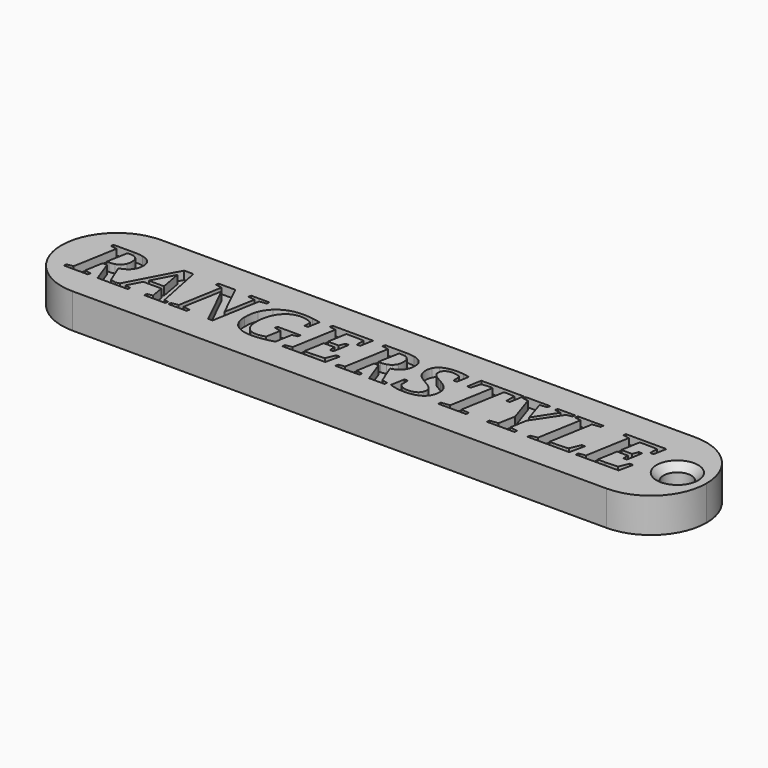
from build123d import *

# Parameters (mm, degrees)
F1_R     = 2
F2_DEPTH = 5
F3_START = 3.8
F3_DEPTH = 25
F4_SIZE  = 1


# Not quite as in the source:
# - ends of sketch curves that miss each other by under 0.0002 mm in the source are joined


with BuildPart() as f2:
    # F1 (on Top) → F2 (new body)
    with BuildSketch(Plane.XY):
        with BuildLine():
            Line((41.2404064533, 8), (-35.7595935467, 8))
            ThreePointArc((-35.7595935467, 8), (-41.4164477962, 5.6568542495), (-43.7595935467, 0))
            ThreePointArc((-43.7595935467, 0), (-41.4164477962, -5.6568542495), (-35.7595935467, -8))
            Line((-35.7595935467, -8), (41.2404064533, -8))
            ThreePointArc((41.2404064533, -8), (46.8972607028, -5.6568542495), (49.2404064533, 0))
            ThreePointArc((49.2404064533, 0), (46.8972607028, 5.6568542495), (41.2404064533, 8))
        make_face()
        with Locations((45.0494252145, 0)):
            Circle(F1_R, mode=Mode.SUBTRACT)
    extrude(amount=F2_DEPTH)

    # F0 (on Top) → F3 (cut)
    with BuildSketch(Plane.XY.offset(F3_START)):
        with BuildLine():
            add(Edge.make_bspline(
                [(-36.2724312993, 3.7303402653), (-35.7735742613, 3.7303402653), (-35.3449268567, 3.6896925164), (-34.9864890067, 3.6083970974)],
                knots=[0, 0, 0, 0, 1, 1, 1, 1], degree=3))
            Line((-36.2724312993, 3.7303402653), (-39.2378577235, 3.7303402653))
            Line((-39.2378577235, 3.7303402653), (-39.3099148564, 3.3257116948))
            Line((-39.3099148564, 3.3257116948), (-38.3842583864, 3.1815979019))
            Line((-38.3842583864, 3.1815979019), (-39.4983718703, -3.1483410183))
            Line((-39.4983718703, -3.1483410183), (-40.4073998198, -3.2979982558))
            Line((-40.4073998198, -3.2979982558), (-40.47391406, -3.7026261956))
            Line((-40.47391406, -3.7026261956), (-36.99854497, -3.7026261956))
            Line((-36.99854497, -3.7026261956), (-36.9320305721, -3.2979982558))
            Line((-36.9320305721, -3.2979982558), (-37.8576874363, -3.1483410183))
            Line((-37.8576874363, -3.1483410183), (-37.3976307265, -0.554285808))
            Line((-37.3976307265, -0.554285808), (-36.7546592649, -0.554285808))
            Line((-36.7546592649, -0.554285808), (-35.601745768, -3.7026261956))
            Line((-35.601745768, -3.7026261956), (-33.4622044537, -3.7026261956))
            Line((-33.4622044537, -3.7026261956), (-33.3846044279, -3.2979982558))
            Line((-33.3846044279, -3.2979982558), (-33.3572007613, -3.2908147575))
            Line((-33.3572007613, -3.2908147575), (-34.1328899849, -3.1483410183))
            Line((-34.1328899849, -3.1483410183), (-35.2470031536, -0.3990857565))
            add(Edge.make_bspline(
                [(-34.5264322969, -0.11085754), (-34.7481465097, -0.2328003137), (-34.9883368216, -0.3288763596), (-35.2470031536, -0.3990857565)],
                knots=[0, 0, 0, 0, 1, 1, 1, 1], degree=3))
            add(Edge.make_bspline(
                [(-33.9444330499, 0.3491998005), (-34.1070230995, 0.1681332577), (-34.3010228485, 0.0147808634), (-34.5264322969, -0.11085754)],
                knots=[0, 0, 0, 0, 1, 1, 1, 1], degree=3))
            add(Edge.make_bspline(
                [(-33.5619757351, 0.9977134454), (-33.654356782, 0.7501327412), (-33.7818426061, 0.5339615), (-33.9444330499, 0.3491998005)],
                knots=[0, 0, 0, 0, 1, 1, 1, 1], degree=3))
            add(Edge.make_bspline(
                [(-33.4234047561, 1.8568559118), (-33.4234047561, 1.5353701809), (-33.4695950825, 1.2489893851), (-33.5619757351, 0.9977134454)],
                knots=[0, 0, 0, 0, 1, 1, 1, 1], degree=3))
            add(Edge.make_bspline(
                [(-33.5896904355, 2.671655236), (-33.4788332896, 2.4388553953), (-33.4234047561, 2.1672556205), (-33.4234047561, 1.8568559118)],
                knots=[0, 0, 0, 0, 1, 1, 1, 1], degree=3))
            add(Edge.make_bspline(
                [(-34.1051752846, 3.253654483), (-33.8723754439, 3.0984548257), (-33.7005471083, 2.9044550767), (-33.5896904355, 2.671655236)],
                knots=[0, 0, 0, 0, 1, 1, 1, 1], degree=3))
            add(Edge.make_bspline(
                [(-34.9864890067, 3.6083970974), (-34.6280511567, 3.5307973082), (-34.3342799686, 3.4125497701), (-34.1051752846, 3.253654483)],
                knots=[0, 0, 0, 0, 1, 1, 1, 1], degree=3))
        make_face()
        with BuildLine():
            add(Edge.make_bspline(
                [(-36.9874593421, 0.0554281393), (-36.6844501044, 0.0554281393), (-36.4128503297, 0.094228231), (-36.1726600178, 0.1718284933)],
                knots=[0, 0, 0, 0, 1, 1, 1, 1], degree=3))
            Line((-36.9874593421, 0.0554281393), (-37.2923160004, 0.0554281393))
            Line((-37.2923160004, 0.0554281393), (-36.7491164509, 3.120626318))
            Line((-36.7491164509, 3.120626318), (-36.3666597669, 3.120626318))
            add(Edge.make_bspline(
                [(-35.3855747633, 2.8046834011), (-35.6072889761, 3.015311986), (-35.9343173632, 3.120626318), (-36.3666597669, 3.120626318)],
                knots=[0, 0, 0, 0, 1, 1, 1, 1], degree=3))
            add(Edge.make_bspline(
                [(-35.0474605907, 1.7681702582), (-35.0474605907, 2.248550803), (-35.1601653149, 2.5940552103), (-35.3855747633, 2.8046834011)],
                knots=[0, 0, 0, 0, 1, 1, 1, 1], degree=3))
            add(Edge.make_bspline(
                [(-35.1804893864, 1.0420559569), (-35.0918034963, 1.2563797774), (-35.0474605907, 1.4984179041), (-35.0474605907, 1.7681702582)],
                knots=[0, 0, 0, 0, 1, 1, 1, 1], degree=3))
            add(Edge.make_bspline(
                [(-35.5629460705, 0.5043992213), (-35.3966603911, 0.6522088805), (-35.2691748035, 0.831427766), (-35.1804893864, 1.0420559569)],
                knots=[0, 0, 0, 0, 1, 1, 1, 1], degree=3))
            add(Edge.make_bspline(
                [(-36.1726600178, 0.1718284933), (-35.932469706, 0.2494282825), (-35.7292317498, 0.3602851919), (-35.5629460705, 0.5043992213)],
                knots=[0, 0, 0, 0, 1, 1, 1, 1], degree=3))
        make_face(mode=Mode.SUBTRACT)
        Polygon((-32.8136908088, -3.1483410183), (-33.3572007613, -3.2908147575), (-33.3180906607, -3.2979982558), (-33.3846044279, -3.7026261956), (-31.2783206278, -3.7026261956), (-31.2007206021, -3.2979982558), (-32.0210627402, -3.1483410183), (-31.0011774085, -1.2249707087), (-28.3849509425, -1.2249707087), (-28.0468367699, -3.1483410183), (-28.8117507687, -3.2979982558), (-28.8893507944, -3.7026261956), (-25.8463238716, -3.7026261956), (-25.7687238458, -3.2979982558), (-26.3728949793, -3.1483410183), (-27.780779809, 3.7913112186), (-29.1110646131, 3.7913112186), align=None)
        Polygon((-30.6907779362, -0.6152567613), (-29.0556358431, 2.4942839288), (-28.4958078518, -0.6152567613), align=None, mode=Mode.SUBTRACT)
        Polygon((-33.3180906607, -3.2979982558), (-33.3572007613, -3.2908147575), (-33.3846044279, -3.2979982558), (-33.4622044537, -3.7026261956), (-33.3846044279, -3.7026261956), align=None)
        with BuildLine():
            add(Edge.make_bspline(
                [(-16.7006159225, -0.8037136964), (-16.7006159225, -0.0609715839), (-16.5805208059, 0.5967802681), (-16.3403304941, 1.1695419387)],
                knots=[0, 0, 0, 0, 1, 1, 1, 1], degree=3))
            add(Edge.make_bspline(
                [(-16.4844442871, -2.0619419193), (-16.6285583165, -1.6887228117), (-16.7006152918, -1.2693134566), (-16.7006159225, -0.8037136964)],
                knots=[0, 0, 0, 0, 1, 1, 1, 1], degree=3))
            add(Edge.make_bspline(
                [(-15.852559084, -3.0097694086), (-16.1297014361, -2.747407841), (-16.3403298635, -2.4314653971), (-16.4844442871, -2.0619419193)],
                knots=[0, 0, 0, 0, 1, 1, 1, 1], degree=3))
            add(Edge.make_bspline(
                [(-14.8215881243, -3.6083977281), (-15.2280641155, -3.4679789342), (-15.571721102, -3.2684361348), (-15.852559084, -3.0097694086)],
                knots=[0, 0, 0, 0, 1, 1, 1, 1], degree=3))
            add(Edge.make_bspline(
                [(-13.4192461084, -3.813483105), (-13.9439696378, -3.813483105), (-14.4114169764, -3.7451212864), (-14.8215881243, -3.6083977281)],
                knots=[0, 0, 0, 0, 1, 1, 1, 1], degree=3))
            add(Edge.make_bspline(
                [(-12.5545608281, -3.7802262214), (-12.8280084178, -3.8023974771), (-13.1162368708, -3.813483105), (-13.4192461084, -3.813483105)],
                knots=[0, 0, 0, 0, 1, 1, 1, 1], degree=3))
            add(Edge.make_bspline(
                [(-11.7563899457, -3.6804549399), (-12.0113615151, -3.7247978455), (-12.277418476, -3.7580549656), (-12.5545608281, -3.7802262214)],
                knots=[0, 0, 0, 0, 1, 1, 1, 1], degree=3))
            add(Edge.make_bspline(
                [(-11.0025622054, -3.5252548884), (-11.246447674, -3.5843786575), (-11.4977236137, -3.6361120343), (-11.7563899457, -3.6804549399)],
                knots=[0, 0, 0, 0, 1, 1, 1, 1], degree=3))
            add(Edge.make_bspline(
                [(-10.2653629069, -3.3146266976), (-10.512943611, -3.3922264869), (-10.7586767368, -3.4624358838), (-11.0025622054, -3.5252548884)],
                knots=[0, 0, 0, 0, 1, 1, 1, 1], degree=3))
            Line((-10.2653629069, -3.3146266976), (-9.8385630807, -0.8979421639))
            Line((-9.8385630807, -0.8979421639), (-9.0847347097, -0.7205708567))
            Line((-9.0847347097, -0.7205708567), (-9.0182209425, -0.3436569865))
            Line((-9.0182209425, -0.3436569865), (-12.3328470095, -0.3436569865))
            Line((-12.3328470095, -0.3436569865), (-12.3993614073, -0.7205708567))
            Line((-12.3993614073, -0.7205708567), (-11.4737045431, -0.8979421639))
            Line((-11.4737045431, -0.8979421639), (-11.8506184132, -3.0042265947))
            add(Edge.make_bspline(
                [(-12.3938185934, -3.1649694601), (-12.1610187527, -3.1095409266), (-11.9799519734, -3.0559599714), (-11.8506184132, -3.0042265947)],
                knots=[0, 0, 0, 0, 1, 1, 1, 1], degree=3))
            add(Edge.make_bspline(
                [(-13.1642747755, -3.2425694858), (-12.879741558, -3.2425694858), (-12.6229228044, -3.2167028368), (-12.3938185934, -3.1649694601)],
                knots=[0, 0, 0, 0, 1, 1, 1, 1], degree=3))
            add(Edge.make_bspline(
                [(-13.9014747047, -3.0984550622), (-13.6797604918, -3.1945313446), (-13.4340271295, -3.2425694858), (-13.1642747755, -3.2425694858)],
                knots=[0, 0, 0, 0, 1, 1, 1, 1], degree=3))
            add(Edge.make_bspline(
                [(-14.4723883238, -2.6661124221), (-14.3134930368, -2.8582649869), (-14.1231885233, -3.002379174), (-13.9014747047, -3.0984550622)],
                knots=[0, 0, 0, 0, 1, 1, 1, 1], degree=3))
            add(Edge.make_bspline(
                [(-14.84375938, -1.9344559375), (-14.7550739629, -2.2263795473), (-14.6312836109, -2.4702650947), (-14.4723883238, -2.6661124221)],
                knots=[0, 0, 0, 0, 1, 1, 1, 1], degree=3))
            add(Edge.make_bspline(
                [(-14.9767881758, -0.9145712364), (-14.9767881758, -1.3025707344), (-14.9324452701, -1.6425323277), (-14.84375938, -1.9344559375)],
                knots=[0, 0, 0, 0, 1, 1, 1, 1], degree=3))
            add(Edge.make_bspline(
                [(-14.7273596568, 0.8646846497), (-14.8936453361, 0.3473519856), (-14.9767881758, -0.2457332834), (-14.9767881758, -0.9145712364)],
                knots=[0, 0, 0, 0, 1, 1, 1, 1], degree=3))
            add(Edge.make_bspline(
                [(-14.0455884976, 2.1617125701), (-14.3301217151, 1.814360348), (-14.5573787419, 1.3820177078), (-14.7273596568, 0.8646846497)],
                knots=[0, 0, 0, 0, 1, 1, 1, 1], degree=3))
            add(Edge.make_bspline(
                [(-13.0589606801, 2.9598834525), (-13.4321793147, 2.7788169098), (-13.7610552801, 2.512759949), (-14.0455884976, 2.1617125701)],
                knots=[0, 0, 0, 0, 1, 1, 1, 1], degree=3))
            add(Edge.make_bspline(
                [(-11.8727902996, 3.2314832273), (-12.2866566831, 3.2314832273), (-12.6820468099, 3.1409499953), (-13.0589606801, 2.9598834525)],
                knots=[0, 0, 0, 0, 1, 1, 1, 1], degree=3))
            add(Edge.make_bspline(
                [(-10.8695334097, 3.0984550622), (-11.165152255, 3.1871404793), (-11.4995711921, 3.2314832273), (-11.8727902996, 3.2314832273)],
                knots=[0, 0, 0, 0, 1, 1, 1, 1], degree=3))
            add(Edge.make_bspline(
                [(-10.0990772275, 2.7270833753), (-10.3134006539, 2.8896738191), (-10.5702193287, 3.0134644077), (-10.8695334097, 3.0984550622)],
                knots=[0, 0, 0, 0, 1, 1, 1, 1], degree=3))
            Line((-10.0990772275, 2.7270833753), (-10.1046206721, 1.7626274442))
            Line((-10.1046206721, 1.7626274442), (-9.6390211484, 1.7626274442))
            Line((-9.6390211484, 1.7626274442), (-9.3341638594, 3.4698261184))
            add(Edge.make_bspline(
                [(-10.564677382, 3.7192546374), (-10.1397253706, 3.6601308684), (-9.7295542227, 3.5769880287), (-9.3341638594, 3.4698261184)],
                knots=[0, 0, 0, 0, 1, 1, 1, 1], degree=3))
            add(Edge.make_bspline(
                [(-11.9670193978, 3.813483105), (-11.4570767319, 3.813483105), (-10.9896293933, 3.7820736421), (-10.564677382, 3.7192546374)],
                knots=[0, 0, 0, 0, 1, 1, 1, 1], degree=3))
            add(Edge.make_bspline(
                [(-13.8349609374, 3.508625816), (-13.2585041102, 3.7118640086), (-12.6358568778, 3.813483105), (-11.9670193978, 3.813483105)],
                knots=[0, 0, 0, 0, 1, 1, 1, 1], degree=3))
            add(Edge.make_bspline(
                [(-15.3370742348, 2.616226466), (-14.9121222234, 3.0079215937), (-14.4114177647, 3.3053880175), (-13.8349609374, 3.508625816)],
                knots=[0, 0, 0, 0, 1, 1, 1, 1], degree=3))
            add(Edge.make_bspline(
                [(-16.3403304941, 1.1695419387), (-16.0964450255, 1.7423036092), (-15.7620262461, 2.2245317324), (-15.3370742348, 2.616226466)],
                knots=[0, 0, 0, 0, 1, 1, 1, 1], degree=3))
        make_face()
        Polygon((-19.4720424399, 3.3257116948), (-18.5020430642, 3.1815979019), (-19.2780426909, -1.2249707087), (-21.68918378, 3.7303402653), (-24.0892392413, 3.7303402653), (-24.1612964531, 3.3257116948), (-23.2356402195, 3.1815979019), (-24.3497533882, -3.1483410183), (-25.3308383917, -3.2979982558), (-25.3973527896, -3.7026261956), (-22.7534116233, -3.7026261956), (-22.6868978561, -3.2979982558), (-23.6568972318, -3.1483410183), (-22.6536403418, 2.4610264145), (-19.6549565611, -3.7026261956), (-19.017528544, -3.7026261956), (-17.8091869078, 3.1815979019), (-16.8281019043, 3.3257116948), (-16.7560446925, 3.7303402653), (-19.3999858588, 3.7303402653), align=None)
        with BuildLine():
            add(Edge.make_bspline(
                [(-2.6328545136, 3.0430262922), (-2.7474064221, 3.0578071557), (-2.882282402, 3.0707403619), (-3.0374824535, 3.0818259898)],
                knots=[0, 0, 0, 0, 1, 1, 1, 1], degree=3))
            Line((-2.6328545136, 3.0430262922), (-2.6661113972, 1.8402268393))
            Line((-2.6661113972, 1.8402268393), (-2.1617115453, 1.8402268393))
            Line((-2.1617115453, 1.8402268393), (-1.8291401866, 3.7303402653))
            Line((-1.8291401866, 3.7303402653), (-7.6602220688, 3.7303402653))
            Line((-7.6602220688, 3.7303402653), (-7.7322792806, 3.3257116948))
            Line((-7.7322792806, 3.3257116948), (-6.806623047, 3.1815979019))
            Line((-6.806623047, 3.1815979019), (-7.9207362156, -3.1483410183))
            Line((-7.9207362156, -3.1483410183), (-8.9018212192, -3.2979982558))
            Line((-8.9018212192, -3.2979982558), (-8.9683356171, -3.7026249343))
            Line((-8.9683356171, -3.7026249343), (-2.7769683066, -3.7026249343))
            Line((-2.7769683066, -3.7026249343), (-2.3113687828, -1.6295980178))
            Line((-2.3113687828, -1.6295980178), (-2.8157686348, -1.6295980178))
            Line((-2.8157686348, -1.6295980178), (-3.386682254, -3.0042253334))
            add(Edge.make_bspline(
                [(-3.6527392148, -3.0374828476), (-3.5344916766, -3.0263968256), (-3.445806023, -3.0153109612), (-3.386682254, -3.0042253334)],
                knots=[0, 0, 0, 0, 1, 1, 1, 1], degree=3))
            add(Edge.make_bspline(
                [(-4.0684534131, -3.0651969173), (-3.9058629693, -3.057806525), (-3.7672915173, -3.0485684755), (-3.6527392148, -3.0374828476)],
                knots=[0, 0, 0, 0, 1, 1, 1, 1], degree=3))
            add(Edge.make_bspline(
                [(-4.6171957765, -3.087368173), (-4.4139575839, -3.0799777807), (-4.2310434627, -3.0725873096), (-4.0684534131, -3.0651969173)],
                knots=[0, 0, 0, 0, 1, 1, 1, 1], degree=3))
            add(Edge.make_bspline(
                [(-5.0405440603, -3.092320995), (-4.892721479, -3.0915084481), (-4.7516053925, -3.0898575075), (-4.6171957765, -3.087368173)],
                knots=[0.3264112981, 0.3264112981, 0.3264112981, 0.3264112981, 1, 1, 1, 1], degree=3))
            add(Edge.make_bspline(
                [(-5.2601666075, -3.0929116176), (-5.1853842502, -3.0929116176), (-5.1121767354, -3.0927147434), (-5.0405440603, -3.092320995)],
                knots=[0, 0, 0, 0, 0.3264112981, 0.3264112981, 0.3264112981, 0.3264112981], degree=3))
            Line((-5.2601666075, -3.0929116176), (-6.2745091254, -3.0929116176))
            Line((-6.2745091254, -3.0929116176), (-5.7701092734, -0.2272566326))
            Line((-5.7701092734, -0.2272566326), (-4.2125672061, -0.2272566326))
            Line((-4.2125672061, -0.2272566326), (-4.1903959503, -1.0697700265))
            Line((-4.1903959503, -1.0697700265), (-3.6970823569, -1.0697700265))
            Line((-3.6970823569, -1.0697700265), (-3.2924537864, 1.2138850808))
            Line((-3.2924537864, 1.2138850808), (-3.7857680105, 1.2138850808))
            Line((-3.7857680105, 1.2138850808), (-4.1017102967, 0.3935429426))
            Line((-4.1017102967, 0.3935429426), (-5.6592523641, 0.3935429426))
            Line((-5.6592523641, 0.3935429426), (-5.1770237678, 3.1206269486))
            Line((-5.1770237678, 3.1206269486), (-4.4121103997, 3.1206269486))
            add(Edge.make_bspline(
                [(-3.9963962013, 3.115083504), (-4.1515962528, 3.1187791337), (-4.290167626, 3.1206269486), (-4.4121103997, 3.1206269486)],
                knots=[0, 0, 0, 0, 1, 1, 1, 1], degree=3))
            add(Edge.make_bspline(
                [(-3.5141676051, 3.1039978761), (-3.6767580489, 3.1113882685), (-3.8375009143, 3.115083504), (-3.9963962013, 3.115083504)],
                knots=[0, 0, 0, 0, 1, 1, 1, 1], degree=3))
            add(Edge.make_bspline(
                [(-3.0374824535, 3.0818259898), (-3.1889872694, 3.0929120118), (-3.3478823199, 3.1003026406), (-3.5141676051, 3.1039978761)],
                knots=[0, 0, 0, 0, 1, 1, 1, 1], degree=3))
        make_face()
        with BuildLine():
            add(Edge.make_bspline(
                [(-3.6527392148, -3.0374828476), (-3.5344916766, -3.0263968256), (-3.445806023, -3.0153109612), (-3.386682254, -3.0042253334)],
                knots=[0, 0, 0, 0, 1, 1, 1, 1], degree=3))
            Line((-3.386682254, -3.0042253334), (-5.0405440603, -3.092320995))
            add(Edge.make_bspline(
                [(-5.0405440603, -3.092320995), (-4.892721479, -3.0915084481), (-4.7516053925, -3.0898575075), (-4.6171957765, -3.087368173)],
                knots=[0.3264112981, 0.3264112981, 0.3264112981, 0.3264112981, 1, 1, 1, 1], degree=3))
            add(Edge.make_bspline(
                [(-4.6171957765, -3.087368173), (-4.4139575839, -3.0799777807), (-4.2310434627, -3.0725873096), (-4.0684534131, -3.0651969173)],
                knots=[0, 0, 0, 0, 1, 1, 1, 1], degree=3))
            add(Edge.make_bspline(
                [(-4.0684534131, -3.0651969173), (-3.9058629693, -3.057806525), (-3.7672915173, -3.0485684755), (-3.6527392148, -3.0374828476)],
                knots=[0, 0, 0, 0, 1, 1, 1, 1], degree=3))
        make_face()
        with BuildLine():
            add(Edge.make_bspline(
                [(2.8822850823, 3.7303402653), (3.3811417261, 3.7303402653), (3.8097888942, 3.6896925164), (4.1682267442, 3.6083970974)],
                knots=[0, 0, 0, 0, 1, 1, 1, 1], degree=3))
            Line((2.8822850823, 3.7303402653), (-0.0831418149, 3.7303402653))
            Line((-0.0831418149, 3.7303402653), (-0.1551990267, 3.3257116948))
            Line((-0.1551990267, 3.3257116948), (0.7704578376, 3.1815979019))
            Line((0.7704578376, 3.1815979019), (-0.3436559617, -3.1483410183))
            Line((-0.3436559617, -3.1483410183), (-1.2526837535, -3.2979982558))
            Line((-1.2526837535, -3.2979982558), (-1.3191981514, -3.7026261956))
            Line((-1.3191981514, -3.7026261956), (2.156170781, -3.7026261956))
            Line((2.156170781, -3.7026261956), (2.2226851789, -3.2979982558))
            Line((2.2226851789, -3.2979982558), (1.2970289453, -3.1483410183))
            Line((1.2970289453, -3.1483410183), (1.7570856551, -0.554285808))
            Line((1.7570856551, -0.554285808), (2.4000564861, -0.554285808))
            Line((2.4000564861, -0.554285808), (3.5529699829, -3.7026261956))
            Line((3.5529699829, -3.7026261956), (5.770111323, -3.7026261956))
            Line((5.770111323, -3.7026261956), (5.8366257209, -3.2979982558))
            Line((5.8366257209, -3.2979982558), (5.0218263966, -3.1483410183))
            Line((5.0218263966, -3.1483410183), (3.9077125973, -0.3990857565))
            add(Edge.make_bspline(
                [(4.628283454, -0.11085754), (4.4065696354, -0.2328003137), (4.1663793235, -0.3288763596), (3.9077125973, -0.3990857565)],
                knots=[0, 0, 0, 0, 1, 1, 1, 1], degree=3))
            add(Edge.make_bspline(
                [(5.2102833317, 0.3491998005), (5.047692888, 0.1681332577), (4.8536929024, 0.0147808634), (4.628283454, -0.11085754)],
                knots=[0, 0, 0, 0, 1, 1, 1, 1], degree=3))
            add(Edge.make_bspline(
                [(5.5927400158, 0.9977134454), (5.5003593631, 0.7501327412), (5.3728737755, 0.5339615), (5.2102833317, 0.3491998005)],
                knots=[0, 0, 0, 0, 1, 1, 1, 1], degree=3))
            add(Edge.make_bspline(
                [(5.7313116255, 1.8568559118), (5.7313116255, 1.5353701809), (5.6851210626, 1.2489893851), (5.5927400158, 0.9977134454)],
                knots=[0, 0, 0, 0, 1, 1, 1, 1], degree=3))
            add(Edge.make_bspline(
                [(5.5650259461, 2.671655236), (5.675883092, 2.4388553953), (5.7313116255, 2.1672556205), (5.7313116255, 1.8568559118)],
                knots=[0, 0, 0, 0, 1, 1, 1, 1], degree=3))
            add(Edge.make_bspline(
                [(5.0495404663, 3.253654483), (5.282340307, 3.0984548257), (5.4541688003, 2.9044550767), (5.5650259461, 2.671655236)],
                knots=[0, 0, 0, 0, 1, 1, 1, 1], degree=3))
            add(Edge.make_bspline(
                [(4.1682267442, 3.6083970974), (4.5266645942, 3.5307973082), (4.8204357823, 3.4125497701), (5.0495404663, 3.253654483)],
                knots=[0, 0, 0, 0, 1, 1, 1, 1], degree=3))
        make_face()
        with BuildLine():
            add(Edge.make_bspline(
                [(2.1672570395, 0.0554281393), (2.4702662772, 0.0554281393), (2.7418660519, 0.094228231), (2.9820563637, 0.1718284933)],
                knots=[0, 0, 0, 0, 1, 1, 1, 1], degree=3))
            Line((2.1672570395, 0.0554281393), (1.8623997505, 0.0554281393))
            Line((1.8623997505, 0.0554281393), (2.4055993, 3.120626318))
            Line((2.4055993, 3.120626318), (2.7880566147, 3.120626318))
            add(Edge.make_bspline(
                [(3.7691416183, 2.8046834011), (3.5474274055, 3.015311986), (3.2203990184, 3.120626318), (2.7880566147, 3.120626318)],
                knots=[0, 0, 0, 0, 1, 1, 1, 1], degree=3))
            add(Edge.make_bspline(
                [(4.1072551603, 1.7681702582), (4.1072551603, 2.248550803), (3.9945506726, 2.5940552103), (3.7691416183, 2.8046834011)],
                knots=[0, 0, 0, 0, 1, 1, 1, 1], degree=3))
            add(Edge.make_bspline(
                [(3.9742269952, 1.0420559569), (4.0629124123, 1.2563797774), (4.1072551603, 1.4984179041), (4.1072551603, 1.7681702582)],
                knots=[0, 0, 0, 0, 1, 1, 1, 1], degree=3))
            add(Edge.make_bspline(
                [(3.5917703111, 0.5043992213), (3.7580555963, 0.6522088805), (3.8855411051, 0.831427766), (3.9742269952, 1.0420559569)],
                knots=[0, 0, 0, 0, 1, 1, 1, 1], degree=3))
            add(Edge.make_bspline(
                [(2.9820563637, 0.1718284933), (3.2222466756, 0.2494282825), (3.4254846318, 0.3602851919), (3.5917703111, 0.5043992213)],
                knots=[0, 0, 0, 0, 1, 1, 1, 1], degree=3))
        make_face(mode=Mode.SUBTRACT)
        with BuildLine():
            add(Edge.make_bspline(
                [(8.6745666362, -3.813483105), (8.1904908558, -3.813483105), (7.7636912661, -3.7728355926), (7.3941677882, -3.6915405678)],
                knots=[0, 0, 0, 0, 1, 1, 1, 1], degree=3))
            add(Edge.make_bspline(
                [(10.0381089545, -3.6582836842), (9.6427190642, -3.7617499647), (9.1882051683, -3.813483105), (8.6745666362, -3.813483105)],
                knots=[0, 0, 0, 0, 1, 1, 1, 1], degree=3))
            add(Edge.make_bspline(
                [(11.0469086585, -3.1982263437), (10.7734610688, -3.4014645364), (10.4371944746, -3.5548170095), (10.0381089545, -3.6582836842)],
                knots=[0, 0, 0, 0, 1, 1, 1, 1], degree=3))
            add(Edge.make_bspline(
                [(11.6677082337, -2.4277701616), (11.5272890456, -2.7344746348), (11.3203558539, -2.9912933884), (11.0469086585, -3.1982263437)],
                knots=[0, 0, 0, 0, 1, 1, 1, 1], degree=3))
            add(Edge.make_bspline(
                [(11.8838792384, -1.3579995044), (11.8838792384, -1.7644754956), (11.8118222631, -2.1210656884), (11.6677082337, -2.4277701616)],
                knots=[0, 0, 0, 0, 1, 1, 1, 1], degree=3))
            add(Edge.make_bspline(
                [(11.7508510734, -0.6318852031), (11.8395364905, -0.8388186313), (11.8838792384, -1.0808566792), (11.8838792384, -1.3579995044)],
                knots=[0, 0, 0, 0, 1, 1, 1, 1], degree=3))
            add(Edge.make_bspline(
                [(11.3961084589, -0.0720572118), (11.5439176451, -0.2346476556), (11.6621651833, -0.4212570123), (11.7508510734, -0.6318852031)],
                knots=[0, 0, 0, 0, 1, 1, 1, 1], degree=3))
            add(Edge.make_bspline(
                [(10.891708607, 0.3658282423), (11.0801655421, 0.2401903118), (11.2482987998, 0.0942284675), (11.3961084589, -0.0720572118)],
                knots=[0, 0, 0, 0, 1, 1, 1, 1], degree=3))
            add(Edge.make_bspline(
                [(10.3207949878, 0.7261136706), (10.5166423152, 0.6152565248), (10.7069469075, 0.4951614083), (10.891708607, 0.3658282423)],
                knots=[0, 0, 0, 0, 1, 1, 1, 1], degree=3))
            add(Edge.make_bspline(
                [(9.749880738, 1.0475987708), (9.9383376731, 0.9441324902), (10.128642423, 0.8369708165), (10.3207949878, 0.7261136706)],
                knots=[0, 0, 0, 0, 1, 1, 1, 1], degree=3))
            add(Edge.make_bspline(
                [(9.2510237, 1.3746273155), (9.3988333591, 1.260075013), (9.5651190385, 1.1510654455), (9.749880738, 1.0475987708)],
                knots=[0, 0, 0, 0, 1, 1, 1, 1], degree=3))
            add(Edge.make_bspline(
                [(8.8962810856, 1.7515411857), (8.9849669757, 1.6148176274), (9.1032145138, 1.4891796181), (9.2510237, 1.3746273155)],
                knots=[0, 0, 0, 0, 1, 1, 1, 1], degree=3))
            add(Edge.make_bspline(
                [(8.7632529205, 2.222684154), (8.7632529205, 2.0453128468), (8.8075956685, 1.888265217), (8.8962810856, 1.7515411857)],
                knots=[0, 0, 0, 0, 1, 1, 1, 1], degree=3))
            add(Edge.make_bspline(
                [(8.8408529462, 2.6051408381), (8.7891195694, 2.4831980644), (8.7632529205, 2.3557125556), (8.7632529205, 2.222684154)],
                knots=[0, 0, 0, 0, 1, 1, 1, 1], degree=3))
            add(Edge.make_bspline(
                [(9.0791958374, 2.9321693829), (8.9720339271, 2.839788336), (8.892586323, 2.7307787686), (8.8408529462, 2.6051408381)],
                knots=[0, 0, 0, 0, 1, 1, 1, 1], degree=3))
            add(Edge.make_bspline(
                [(9.4949094051, 3.1538832016), (9.3249284901, 3.0984546681), (9.1863573535, 3.0245500356), (9.0791958374, 2.9321693829)],
                knots=[0, 0, 0, 0, 1, 1, 1, 1], degree=3))
            add(Edge.make_bspline(
                [(10.1046233524, 3.2370260412), (9.8681282761, 3.2370260412), (9.66489032, 3.2093117351), (9.4949094051, 3.1538832016)],
                knots=[0, 0, 0, 0, 1, 1, 1, 1], degree=3))
            add(Edge.make_bspline(
                [(10.7642232558, 3.1427975737), (10.5683754555, 3.2056165783), (10.348508821, 3.2370260412), (10.1046233524, 3.2370260412)],
                knots=[0, 0, 0, 0, 1, 1, 1, 1], degree=3))
            add(Edge.make_bspline(
                [(11.2741652911, 2.8933690547), (11.1337464972, 3.0005309649), (10.9637658188, 3.0836738046), (10.7642232558, 3.1427975737)],
                knots=[0, 0, 0, 0, 1, 1, 1, 1], degree=3))
            Line((11.2741652911, 2.8933690547), (11.3129656193, 1.8069699557))
            Line((11.3129656193, 1.8069699557), (11.8062792127, 1.8069699557))
            Line((11.8062792127, 1.8069699557), (12.1166793156, 3.5751402138))
            add(Edge.make_bspline(
                [(11.2187371517, 3.7469687071), (11.5476128807, 3.7026258015), (11.8469269616, 3.6453496108), (12.1166793156, 3.5751402138)],
                knots=[0, 0, 0, 0, 1, 1, 1, 1], degree=3))
            add(Edge.make_bspline(
                [(10.2542805899, 3.813483105), (10.5683754555, 3.813483105), (10.8898610286, 3.7913116127), (11.2187371517, 3.7469687071)],
                knots=[0, 0, 0, 0, 1, 1, 1, 1], degree=3))
            add(Edge.make_bspline(
                [(9.0348526952, 3.6859971232), (9.3932905452, 3.7709877777), (9.7997664576, 3.813483105), (10.2542805899, 3.813483105)],
                knots=[0, 0, 0, 0, 1, 1, 1, 1], degree=3))
            add(Edge.make_bspline(
                [(8.1202820895, 3.2979976252), (8.3715580292, 3.4716736968), (8.6764148452, 3.6010068628), (9.0348526952, 3.6859971232)],
                knots=[0, 0, 0, 0, 1, 1, 1, 1], degree=3))
            add(Edge.make_bspline(
                [(7.5493678397, 2.6439405357), (7.6823966354, 2.9063024974), (7.8727013854, 3.1243215535), (8.1202820895, 3.2979976252)],
                knots=[0, 0, 0, 0, 1, 1, 1, 1], degree=3))
            add(Edge.make_bspline(
                [(7.3553680907, 1.723827116), (7.3553680907, 2.0785697304), (7.4200346737, 2.3852742037), (7.5493678397, 2.6439405357)],
                knots=[0, 0, 0, 0, 1, 1, 1, 1], degree=3))
            add(Edge.make_bspline(
                [(7.4883968864, 0.9699993757), (7.3997109963, 1.1843228021), (7.3553680907, 1.435598663), (7.3553680907, 1.723827116)],
                knots=[0, 0, 0, 0, 1, 1, 1, 1], degree=3))
            add(Edge.make_bspline(
                [(7.8375966869, 0.3990851259), (7.6934822633, 0.5653708052), (7.5770823035, 0.7556755552), (7.4883968864, 0.9699993757)],
                knots=[0, 0, 0, 0, 1, 1, 1, 1], degree=3))
            add(Edge.make_bspline(
                [(8.3364530943, -0.0443431421), (8.1516913948, 0.0849900239), (7.9854058731, 0.2327994466), (7.8375966869, 0.3990851259)],
                knots=[0, 0, 0, 0, 1, 1, 1, 1], degree=3))
            add(Edge.make_bspline(
                [(8.9018245301, -0.3990857565), (8.7096719653, -0.2882286107), (8.5212147938, -0.1699810726), (8.3364530943, -0.0443431421)],
                knots=[0, 0, 0, 0, 1, 1, 1, 1], degree=3))
            add(Edge.make_bspline(
                [(9.4727381493, -0.7205708567), (9.2879764498, -0.6134093406), (9.0976718575, -0.5062476668), (8.9018245301, -0.3990857565)],
                knots=[0, 0, 0, 0, 1, 1, 1, 1], degree=3))
            add(Edge.make_bspline(
                [(9.9660523734, -1.0586850293), (9.8219379498, -0.9367422556), (9.6574998488, -0.8240375314), (9.4727381493, -0.7205708567)],
                knots=[0, 0, 0, 0, 1, 1, 1, 1], degree=3))
            add(Edge.make_bspline(
                [(10.3207949878, -1.4577707859), (10.2321090977, -1.3099611267), (10.1138615596, -1.1769325675), (9.9660523734, -1.0586850293)],
                knots=[0, 0, 0, 0, 1, 1, 1, 1], degree=3))
            add(Edge.make_bspline(
                [(10.4538231529, -1.9787990796), (10.4538231529, -1.7792561225), (10.4094804049, -1.605579972), (10.3207949878, -1.4577707859)],
                knots=[0, 0, 0, 0, 1, 1, 1, 1], degree=3))
            add(Edge.make_bspline(
                [(10.3540518714, -2.4831983009), (10.4205660328, -2.3279986436), (10.4538231529, -2.1598656224), (10.4538231529, -1.9787990796)],
                knots=[0, 0, 0, 0, 1, 1, 1, 1], degree=3))
            add(Edge.make_bspline(
                [(10.0491945824, -2.8878268714), (10.1859186137, -2.7732745688), (10.2875377101, -2.6383983524), (10.3540518714, -2.4831983009)],
                knots=[0, 0, 0, 0, 1, 1, 1, 1], degree=3))
            add(Edge.make_bspline(
                [(9.5226241054, -3.1594266461), (9.7369475318, -3.0929124848), (9.9124710241, -3.002379174), (10.0491945824, -2.8878268714)],
                knots=[0, 0, 0, 0, 1, 1, 1, 1], degree=3))
            add(Edge.make_bspline(
                [(8.7687957344, -3.2536551137), (9.0607193442, -3.2536551137), (9.3119955204, -3.2222456508), (9.5226241054, -3.1594266461)],
                knots=[0, 0, 0, 0, 1, 1, 1, 1], degree=3))
            add(Edge.make_bspline(
                [(8.3253674664, -3.2093126022), (8.4694814958, -3.2388742502), (8.6172909185, -3.2536551137), (8.7687957344, -3.2536551137)],
                knots=[0, 0, 0, 0, 1, 1, 1, 1], degree=3))
            add(Edge.make_bspline(
                [(7.9207388959, -3.0762838065), (8.0463772993, -3.13171234), (8.181253437, -3.1760553244), (8.3253674664, -3.2093126022)],
                knots=[0, 0, 0, 0, 1, 1, 1, 1], degree=3))
            add(Edge.make_bspline(
                [(7.57708254, -2.8711984296), (7.6805488206, -2.9487982188), (7.7951009655, -3.0171600374), (7.9207388959, -3.0762838065)],
                knots=[0, 0, 0, 0, 1, 1, 1, 1], degree=3))
            add(Edge.make_bspline(
                [(7.3331968349, -2.6162270967), (7.3960158396, -2.7086077493), (7.4773110221, -2.7935981674), (7.57708254, -2.8711984296)],
                knots=[0, 0, 0, 0, 1, 1, 1, 1], degree=3))
            Line((7.3331968349, -2.6162270967), (7.3276533904, -1.4245132716))
            Line((7.3276533904, -1.4245132716), (6.8398819802, -1.4245132716))
            Line((6.8398819802, -1.4245132716), (6.4851393658, -3.419940793))
            add(Edge.make_bspline(
                [(7.3941677882, -3.6915405678), (7.0283391518, -3.6065503074), (6.7253296776, -3.5160170754), (6.4851393658, -3.419940793)],
                knots=[0, 0, 0, 0, 1, 1, 1, 1], degree=3))
        make_face()
        with BuildLine():
            add(Edge.make_bspline(
                [(15.5698763616, 3.1427975737), (15.4848857071, 3.1427975737), (15.3851141891, 3.1391023381), (15.2705618865, 3.1317119458)],
                knots=[0, 0, 0, 0, 1, 1, 1, 1], degree=3))
            Line((15.5698763616, 3.1427975737), (15.9079905342, 3.1427975737))
            Line((15.9079905342, 3.1427975737), (14.7994195488, -3.1483410183))
            Line((14.7994195488, -3.1483410183), (13.591077282, -3.2979982558))
            Line((13.591077282, -3.2979982558), (13.5245635148, -3.7026261956))
            Line((13.5245635148, -3.7026261956), (17.5265035548, -3.7026261956))
            Line((17.5265035548, -3.7026261956), (17.5930179527, -3.2979982558))
            Line((17.5930179527, -3.2979982558), (16.4401044559, -3.1483410183))
            Line((16.4401044559, -3.1483410183), (17.5486748106, 3.1317119458))
            Line((17.5486748106, 3.1317119458), (17.8757033553, 3.1317119458))
            add(Edge.make_bspline(
                [(18.1750171997, 3.120626318), (18.0604648972, 3.1280167103), (17.9606936157, 3.1317119458), (17.8757033553, 3.1317119458)],
                knots=[0, 0, 0, 0, 1, 1, 1, 1], degree=3))
            add(Edge.make_bspline(
                [(18.5297598142, 3.0984550622), (18.411512276, 3.1095406901), (18.2932647379, 3.1169310824), (18.1750171997, 3.120626318)],
                knots=[0, 0, 0, 0, 1, 1, 1, 1], degree=3))
            add(Edge.make_bspline(
                [(18.8623318035, 3.0707403619), (18.7588667843, 3.0818259898), (18.6480094808, 3.0910641969), (18.5297598142, 3.0984550622)],
                knots=[0, 0, 0, 0, 1, 1, 1, 1], degree=3))
            add(Edge.make_bspline(
                [(19.1228421665, 3.0319406643), (19.0563292664, 3.0467215278), (18.9694924525, 3.059654734), (18.8623318035, 3.0707403619)],
                knots=[0, 0, 0, 0, 1, 1, 1, 1], degree=3))
            Line((19.1228421665, 3.0319406643), (19.0507899999, 1.6517699042))
            Line((19.0507899999, 1.6517699042), (19.5385563648, 1.6517699042))
            Line((19.5385563648, 1.6517699042), (19.9043858684, 3.7303402653))
            Line((19.9043858684, 3.7303402653), (13.7906204756, 3.7303402653))
            Line((13.7906204756, 3.7303402653), (13.4247922333, 1.6517699042))
            Line((13.4247922333, 1.6517699042), (13.9070201989, 1.6517699042))
            Line((13.9070201989, 1.6517699042), (14.3227343972, 3.0319406643))
            add(Edge.make_bspline(
                [(14.588791358, 3.0707403619), (14.4816294478, 3.059654734), (14.3929437942, 3.0467215278), (14.3227343972, 3.0319406643)],
                knots=[0, 0, 0, 0, 1, 1, 1, 1], degree=3))
            add(Edge.make_bspline(
                [(14.9213620861, 3.1095406901), (14.8068097835, 3.0984550622), (14.6959528741, 3.0855216195), (14.588791358, 3.0707403619)],
                knots=[0, 0, 0, 0, 1, 1, 1, 1], degree=3))
            add(Edge.make_bspline(
                [(15.2705618865, 3.1317119458), (15.156009584, 3.1280163161), (15.0396096242, 3.1206259238), (14.9213620861, 3.1095406901)],
                knots=[0, 0, 0, 0, 1, 1, 1, 1], degree=3))
        make_face()
        Polygon((23.4296445407, -3.1483410183), (23.8730696555, -0.6651427174), (26.4560373459, 3.1815979019), (27.2708417154, 3.3257116948), (27.342893882, 3.7303402653), (24.8153543309, 3.7303402653), (24.7432958578, 3.3257116948), (25.6246152558, 3.1815979019), (23.607015848, 0.0997712815), (22.6203836159, 3.1815979019), (23.6458136535, 3.3257116948), (23.7178721266, 3.7303402653), (20.1926134543, 3.7303402653), (20.1205612877, 3.3257116948), (20.9298159061, 3.1815979019), (22.2268431959, -0.698399601), (21.7889552192, -3.1483410183), (20.5806167362, -3.2979982558), (20.5141017077, -3.7026261956), (24.5160398558, -3.7026261956), (24.5825548843, -3.2979982558), align=None)
        with BuildLine():
            add(Edge.make_bspline(
                [(29.7096924596, -3.115083504), (29.9018484142, -3.115083504), (30.1069348159, -3.1113882685), (30.3249517435, -3.1039978761)],
                knots=[0, 0, 0, 0, 1, 1, 1, 1], degree=3))
            Line((29.7096924596, -3.115083504), (29.0833525931, -3.115083504))
            Line((29.0833525931, -3.115083504), (30.1919216865, 3.1815979019))
            Line((30.1919216865, 3.1815979019), (31.3115776691, 3.3257116948))
            Line((31.3115776691, 3.3257116948), (31.3836361422, 3.7303402653))
            Line((31.3836361422, 3.7303402653), (27.7087233856, 3.7303402653))
            Line((27.7087233856, 3.7303402653), (27.6366649125, 3.3257116948))
            Line((27.6366649125, 3.3257116948), (28.556782116, 3.1815979019))
            Line((28.556782116, 3.1815979019), (27.442669578, -3.1483410183))
            Line((27.442669578, -3.1483410183), (26.4615807905, -3.2979982558))
            Line((26.4615807905, -3.2979982558), (26.395065762, -3.7026261956))
            Line((26.395065762, -3.7026261956), (32.4090661799, -3.7026261956))
            Line((32.4090661799, -3.7026261956), (32.9023759894, -1.4577707859))
            Line((32.9023759894, -1.4577707859), (32.4367770963, -1.4577707859))
            Line((32.4367770963, -1.4577707859), (31.7882634514, -3.0042265947))
            add(Edge.make_bspline(
                [(31.4723249491, -3.0430269229), (31.6238289766, -3.0282456653), (31.7291418107, -3.0153122225), (31.7882634514, -3.0042265947)],
                knots=[0, 0, 0, 0, 1, 1, 1, 1], degree=3))
            add(Edge.make_bspline(
                [(30.9512916101, -3.0762838065), (31.1471389375, -3.0651981786), (31.3208167434, -3.0541125507), (31.4723249491, -3.0430269229)],
                knots=[0, 0, 0, 0, 1, 1, 1, 1], degree=3))
            add(Edge.make_bspline(
                [(30.3249517435, -3.1039978761), (30.5466643009, -3.0966074838), (30.7554442827, -3.0873694343), (30.9512916101, -3.0762838065)],
                knots=[0, 0, 0, 0, 1, 1, 1, 1], degree=3))
        make_face()
        with BuildLine():
            add(Edge.make_bspline(
                [(39.6702028862, 3.0430262922), (39.5556509778, 3.0578071557), (39.4207752344, 3.0707403619), (39.2655755771, 3.0818259898)],
                knots=[0, 0, 0, 0, 1, 1, 1, 1], degree=3))
            Line((39.6702028862, 3.0430262922), (39.6369485252, 1.8402268393))
            Line((39.6369485252, 1.8402268393), (40.1413452239, 1.8402268393))
            Line((40.1413452239, 1.8402268393), (40.47391406, 3.7303402653))
            Line((40.47391406, 3.7303402653), (34.6428347005, 3.7303402653))
            Line((34.6428347005, 3.7303402653), (34.5707762274, 3.3257116948))
            Line((34.5707762274, 3.3257116948), (35.4964368755, 3.1815979019))
            Line((35.4964368755, 3.1815979019), (34.382318031, -3.1483410183))
            Line((34.382318031, -3.1483410183), (33.40123555, -3.2979982558))
            Line((33.40123555, -3.2979982558), (33.3347205215, -3.7026249343))
            Line((33.3347205215, -3.7026249343), (39.52608594, -3.7026249343))
            Line((39.52608594, -3.7026249343), (39.9916911397, -1.6295980178))
            Line((39.9916911397, -1.6295980178), (39.4872881344, -1.6295980178))
            Line((39.4872881344, -1.6295980178), (38.9163764072, -3.0042253334))
            add(Edge.make_bspline(
                [(38.6503162931, -3.0374828476), (38.7685638313, -3.0263968256), (38.8572505097, -3.0153109612), (38.9163764072, -3.0042253334)],
                knots=[0, 0, 0, 0, 1, 1, 1, 1], degree=3))
            add(Edge.make_bspline(
                [(38.2346020948, -3.0651969173), (38.3971930116, -3.057806525), (38.5357643847, -3.0485684755), (38.6503162931, -3.0374828476)],
                knots=[0, 0, 0, 0, 1, 1, 1, 1], degree=3))
            add(Edge.make_bspline(
                [(37.6858641459, -3.087368173), (37.8890985547, -3.0799777807), (38.072011178, -3.0725873096), (38.2346020948, -3.0651969173)],
                knots=[0, 0, 0, 0, 1, 1, 1, 1], degree=3))
            add(Edge.make_bspline(
                [(37.2625141534, -3.0923209886), (37.4103379363, -3.0915084395), (37.5514546165, -3.0898575009), (37.6858641459, -3.087368173)],
                knots=[0.3264130623, 0.3264130623, 0.3264130623, 0.3264130623, 1, 1, 1, 1], degree=3))
            add(Edge.make_bspline(
                [(37.0428876391, -3.0929116176), (37.1176714813, -3.0929116176), (37.1908803212, -3.0927147413), (37.2625141534, -3.0923209886)],
                knots=[0, 0, 0, 0, 0.3264130623, 0.3264130623, 0.3264130623, 0.3264130623], degree=3))
            Line((37.0428876391, -3.0929116176), (36.0285507971, -3.0929116176))
            Line((36.0285507971, -3.0929116176), (36.5329474958, -0.2272566326))
            Line((36.5329474958, -0.2272566326), (38.0904914551, -0.2272566326))
            Line((38.0904914551, -0.2272566326), (38.1126589269, -1.0697700265))
            Line((38.1126589269, -1.0697700265), (38.605975043, -1.0697700265))
            Line((38.605975043, -1.0697700265), (39.0106023522, 1.2138850808))
            Line((39.0106023522, 1.2138850808), (38.5172862361, 1.2138850808))
            Line((38.5172862361, 1.2138850808), (38.2013477338, 0.3935429426))
            Line((38.2013477338, 0.3935429426), (36.6438037745, 0.3935429426))
            Line((36.6438037745, 0.3935429426), (37.1260330014, 3.1206269486))
            Line((37.1260330014, 3.1206269486), (37.8909463696, 3.1206269486))
            add(Edge.make_bspline(
                [(38.3066605679, 3.115083504), (38.1514609106, 3.1187791337), (38.0128895374, 3.1206269486), (37.8909463696, 3.1206269486)],
                knots=[0, 0, 0, 0, 1, 1, 1, 1], degree=3))
            add(Edge.make_bspline(
                [(38.7888897948, 3.1039978761), (38.626298878, 3.1113882685), (38.4655558549, 3.115083504), (38.3066605679, 3.115083504)],
                knots=[0, 0, 0, 0, 1, 1, 1, 1], degree=3))
            add(Edge.make_bspline(
                [(39.2655755771, 3.0818259898), (39.1140715495, 3.0929120118), (38.9551763413, 3.1003026406), (38.7888897948, 3.1039978761)],
                knots=[0, 0, 0, 0, 1, 1, 1, 1], degree=3))
        make_face()
        with BuildLine():
            add(Edge.make_bspline(
                [(38.6503162931, -3.0374828476), (38.7685638313, -3.0263968256), (38.8572505097, -3.0153109612), (38.9163764072, -3.0042253334)],
                knots=[0, 0, 0, 0, 1, 1, 1, 1], degree=3))
            Line((38.9163764072, -3.0042253334), (37.2625141534, -3.0923209886))
            add(Edge.make_bspline(
                [(37.2625141534, -3.0923209886), (37.4103379363, -3.0915084395), (37.5514546165, -3.0898575009), (37.6858641459, -3.087368173)],
                knots=[0.3264130623, 0.3264130623, 0.3264130623, 0.3264130623, 1, 1, 1, 1], degree=3))
            add(Edge.make_bspline(
                [(37.6858641459, -3.087368173), (37.8890985547, -3.0799777807), (38.072011178, -3.0725873096), (38.2346020948, -3.0651969173)],
                knots=[0, 0, 0, 0, 1, 1, 1, 1], degree=3))
            add(Edge.make_bspline(
                [(38.2346020948, -3.0651969173), (38.3971930116, -3.057806525), (38.5357643847, -3.0485684755), (38.6503162931, -3.0374828476)],
                knots=[0, 0, 0, 0, 1, 1, 1, 1], degree=3))
        make_face()
    extrude(amount=F3_DEPTH, mode=Mode.SUBTRACT)

    # F4
    f4_edges = [f2.edges().sort_by_distance(p)[0] for p in [
        (43.049425, 0, 5),
        (43.049425, 0, 0),
    ]]
    chamfer(f4_edges, length=F4_SIZE)


solid = f2.part
